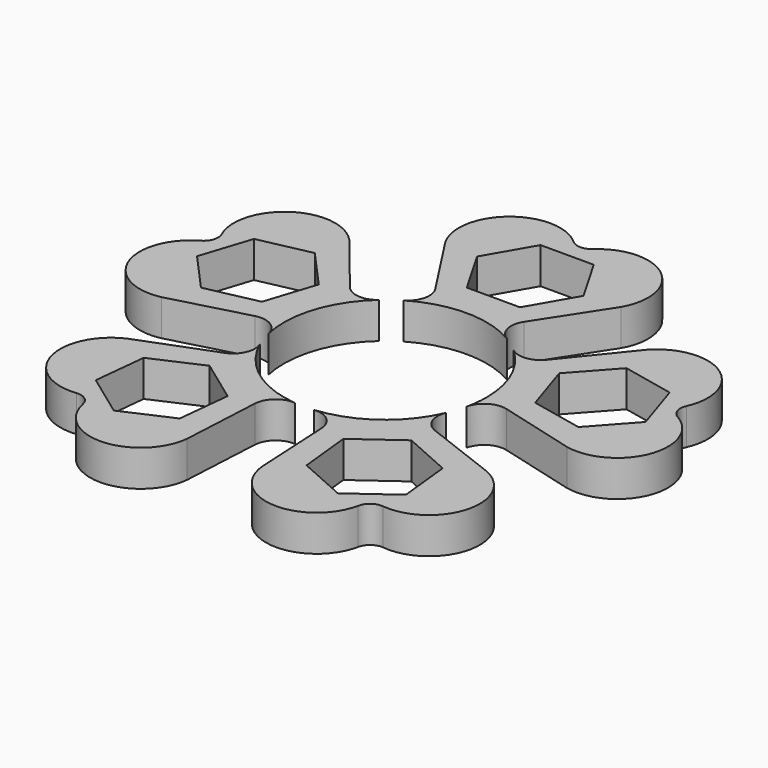
from build123d import *

# Parameters (mm, degrees)
F1_DEPTH = 5


# Not quite as in the source:
# - a feature names something its author has since deleted; it is built from what else it names


with BuildPart() as f1:
    # F0 (on Top) → F1 (new body)
    with BuildSketch(Plane.XY):
        with BuildLine():
            ThreePointArc((-13.665469042, -3.0319204432), (-13.3159762762, 4.3418317), (-9.2645390994, 10.5127491897))
            ThreePointArc((-9.2645390994, 10.5127491897), (-11.4998669549, 9.7726015122), (-13.5809814233, 10.8741784618))
            Line((-13.5809814233, 10.8741784618), (-20.506494271, 19.426474585))
            ThreePointArc((-20.506494271, 19.426474585), (-29.538567909, 20.601795911), (-32.0861364699, 11.8571044442))
            ThreePointArc((-32.0861364699, 11.8571044442), (-32.0062029861, 10.4146544851), (-32.9187213461, 9.2946716776))
            ThreePointArc((-32.9187213461, 9.2946716776), (-35.997695766, 0.7226444411), (-27.9997581563, -3.6354203143))
            Line((-27.9997581563, -3.6354203143), (-17.3699870332, -0.7871817262))
            ThreePointArc((-17.3699870332, -0.7871817262), (-15.0388393758, -1.1192356462), (-13.665469042, -3.0319204432))
        make_face()
        Polygon((-28.6916231536, 13.1985965214), (-21.5082094645, 14.7254782362), (-16.5941842664, 9.267900353), (-18.8635727573, 2.2834407549), (-26.0469864464, 0.7565590401), (-30.9610116446, 6.2141369233), align=None, mode=Mode.SUBTRACT)
    extrude(amount=F1_DEPTH)


with BuildPart() as f1b:
    # F0 (on Top) → F1, piece 2 (new body)
    with BuildSketch(Plane.XY):
        with BuildLine():
            ThreePointArc((-1.3253227589, -13.9216462393), (-8.2301785802, -11.3106441425), (-12.847106931, -5.5505800398))
            ThreePointArc((-12.847106931, -5.5505800398), (-12.8339389546, -7.9052213736), (-14.5247006287, -9.5440728519))
            Line((-14.5247006287, -9.5440728519), (-24.7985187507, -13.4878221314))
            ThreePointArc((-24.7985187507, -13.4878221314), (-28.7073800051, -21.7146403569), (-21.1779261823, -26.8397803113))
            ThreePointArc((-21.1779261823, -26.8397803113), (-19.7813739443, -27.2095006015), (-18.998190678, -28.4234508549))
            ThreePointArc((-18.998190678, -28.4234508549), (-11.7971637379, -34.0006316328), (-5.1808992125, -27.7408570242))
            Line((-5.1808992125, -27.7408570242), (-4.6049551583, -16.7511898031))
            ThreePointArc((-4.6049551583, -16.7511898031), (-3.5687888714, -14.6367469374), (-1.3253227589, -13.9216462393))
        make_face()
        Polygon((-21.4047986615, -23.1968624525), (-20.6371525584, -15.8931976559), (-13.9281702523, -12.906166284), (-7.9868340493, -17.2227997087), (-8.7544801524, -24.5264645053), (-15.4634624585, -27.5134958771), align=None, mode=Mode.SUBTRACT)
    extrude(amount=F1_DEPTH)


with BuildPart() as f1c:
    # F0 (on Top) → F1, piece 3 (new body)
    with BuildSketch(Plane.XY):
        with BuildLine():
            ThreePointArc((7.1196691813, 12.0693664265), (5.7249926142, 13.9665713389), (6.1295548123, 16.2862348132))
            Line((6.1295548123, 16.2862348132), (12.1231706049, 25.5155937788))
            ThreePointArc((12.1231706049, 25.5155937788), (10.4499033622, 34.4688005315), (1.34596558, 34.1894239382))
            ThreePointArc((1.34596558, 34.1894239382), (-0.0011850481, 33.6676611266), (-1.3483356762, 34.1894239382))
            ThreePointArc((-1.3483356762, 34.1894239382), (-10.4522734584, 34.4688005315), (-12.1255407011, 25.5155937788))
            Line((-12.1255407011, 25.5155937788), (-6.1319249085, 16.2862348132))
            ThreePointArc((-6.1319249085, 16.2862348132), (-5.7273627104, 13.9665713389), (-7.1220392775, 12.0693664265))
            ThreePointArc((-7.1220392775, 12.0693664265), (-0.0011850481, 14.0155937788), (7.1196691813, 12.0693664265))
        make_face()
        Polygon((-7.3450804722, 25.0155937788), (-3.6731327602, 31.3755937788), (3.6707626639, 31.3755937788), (7.342710376, 25.0155937788), (3.6707626639, 18.6555937788), (-3.6731327602, 18.6555937788), align=None, mode=Mode.SUBTRACT)
    extrude(amount=F1_DEPTH)


with BuildPart() as f1d:
    # F0 (on Top) → F1, piece 4 (new body)
    with BuildSketch(Plane.XY):
        with BuildLine():
            ThreePointArc((14.5223305325, -9.5440728519), (12.8315688584, -7.9052213736), (12.8447368348, -5.5505800398))
            ThreePointArc((12.8447368348, -5.5505800398), (8.227808484, -11.3106441425), (1.3229526627, -13.9216462393))
            ThreePointArc((1.3229526627, -13.9216462393), (3.5664187752, -14.6367469374), (4.6025850621, -16.7511898031))
            Line((4.6025850621, -16.7511898031), (5.1785291162, -27.7408570242))
            ThreePointArc((5.1785291162, -27.7408570242), (11.7947936417, -34.0006316328), (18.9958205818, -28.4234508549))
            ThreePointArc((18.9958205818, -28.4234508549), (19.7790038481, -27.2095006015), (21.1755560861, -26.8397803113))
            ThreePointArc((21.1755560861, -26.8397803113), (28.7050099089, -21.7146403569), (24.7961486545, -13.4878221314))
            Line((24.7961486545, -13.4878221314), (14.5223305325, -9.5440728519))
        make_face()
        Polygon((7.9844639531, -17.2227997087), (13.9258001561, -12.906166284), (20.6347824622, -15.8931976559), (21.4024285653, -23.1968624525), (15.4610923623, -27.5134958771), (8.7521100562, -24.5264645053), align=None, mode=Mode.SUBTRACT)
    extrude(amount=F1_DEPTH)


with BuildPart() as f1e:
    # F0 (on Top) → F1, piece 5 (new body)
    with BuildSketch(Plane.XY):
        with BuildLine():
            ThreePointArc((13.5786113271, 10.8741784618), (11.4974968587, 9.7726015122), (9.2621690031, 10.5127491897))
            ThreePointArc((9.2621690031, 10.5127491897), (12.7598289539, 5.7737637694), (13.9988149519, 0.0155937788))
            ThreePointArc((13.9988149519, 0.0155937788), (13.9146328566, -1.5173811207), (13.6630989458, -3.0319204432))
            ThreePointArc((13.6630989458, -3.0319204432), (15.0364692796, -1.1192356462), (17.367616937, -0.7871817262))
            Line((17.367616937, -0.7871817262), (27.99738806, -3.6354203143))
            ThreePointArc((27.99738806, -3.6354203143), (35.9953256698, 0.7226444411), (32.9163512498, 9.2946716776))
            ThreePointArc((32.9163512498, 9.2946716776), (32.0038328898, 10.4146544851), (32.0837663737, 11.8571044442))
            ThreePointArc((32.0837663737, 11.8571044442), (29.5361978128, 20.601795911), (20.5041241748, 19.426474585))
            Line((20.5041241748, 19.426474585), (13.5786113271, 10.8741784618))
        make_face()
        Polygon((18.8612026611, 2.2834407549), (16.5918141702, 9.267900353), (21.5058393683, 14.7254782362), (28.6892530574, 13.1985965214), (30.9586415484, 6.2141369233), (26.0446163502, 0.7565590401), align=None, mode=Mode.SUBTRACT)
    extrude(amount=F1_DEPTH)


solid = Compound([f1.part, f1b.part, f1c.part, f1d.part, f1e.part])
